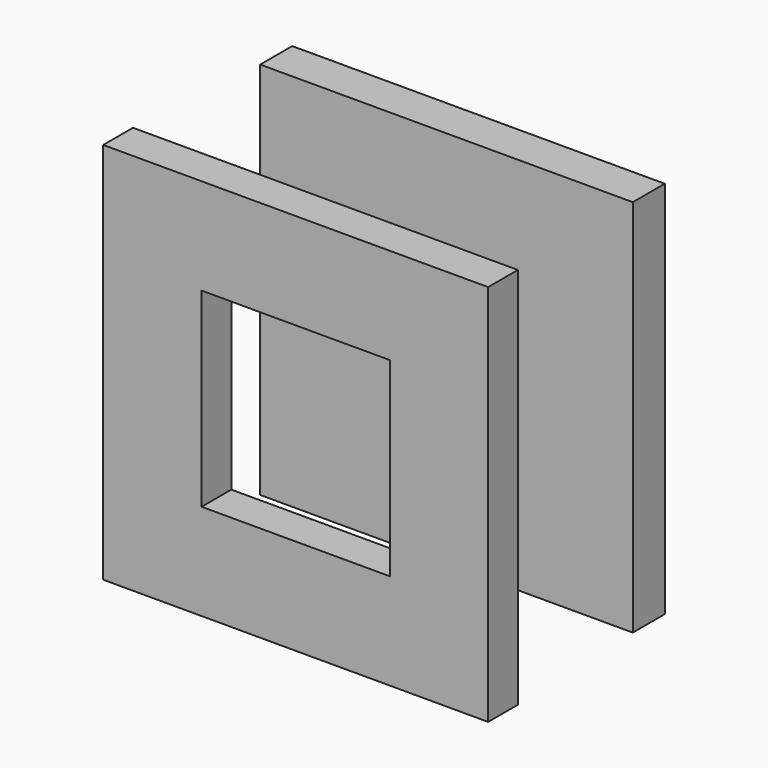
from build123d import *

# Parameters (mm, degrees)
F0_W     = 51.8050342798
F0_H     = 51.5172313899
F0_W_2   = 25.3269076347
F0_H_2   = 25.6147123873
F1_DEPTH = 5
F3_W     = 50.1393936574
F3_H     = 5.3821932524
F4_DEPTH = 21
F5_DEPTH = 30


# Not quite as in the source:
# - the program builds the solid bodies; features that only make, move or delete a surface that nothing else refers to are left out


with BuildPart() as f1:
    # F0 (on Front) → F1 (new body)
    with BuildSketch(Plane.XZ):
        with Locations((3.0219592154, -4.3170871213)):
            Rectangle(F0_W, F0_H)
        with Locations((3.021961078, -4.31708619)):
            Rectangle(F0_W_2, F0_H_2, mode=Mode.SUBTRACT)
    extrude(amount=F1_DEPTH)


with BuildPart() as f4:
    # F3 (on Top) → F4 (new body)
    with BuildSketch(Plane.XY):
        with Locations((3.1160078943, 22.9451442137)):
            Rectangle(F3_W, F3_H)
    extrude(amount=F4_DEPTH)

    # F5 (add): a face of the model
    f5_faces = [f4.faces().sort_by_distance(p)[0] for p in [
        (3.1160078943, 22.9451442137, 0),
    ]]
    extrude(f5_faces, amount=F5_DEPTH)


solid = Compound([f1.part, f4.part])
